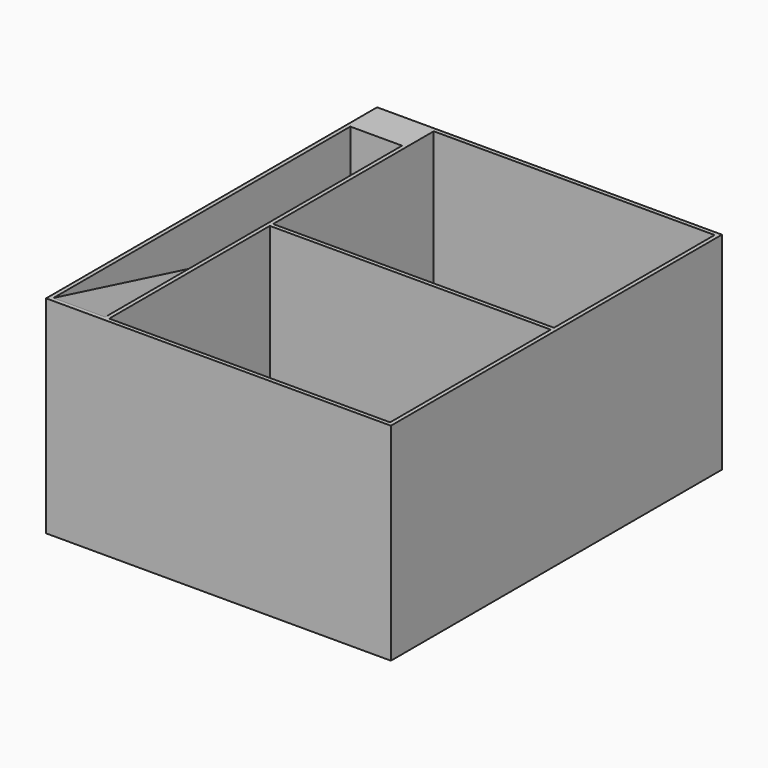
from build123d import *

# Parameters (mm, degrees)
F0_W      = 127
F0_H      = 152.4
F1_DEPTH  = 76.2
F2_T      = -1.4986
F3_W      = 1.4986
F3_H      = 149.4028
F5_DEPTH  = 74.7014
F6_DEPTH  = 19.05
F8_DEPTH  = 19.05
F9_W      = 103.4542
F9_H      = 1.4986
F10_DEPTH = 74.7014


# Not quite as in the source:
# - an extrude ends at something that could not be found from the text; its depth is read off the source's solid


with BuildPart() as f1:
    # F0 (on Top) → F1 (new body)
    with BuildSketch(Plane.XY):
        Rectangle(F0_W, F0_H)
    extrude(amount=F1_DEPTH)

    # F2
    f2_openings = [f1.faces().sort_by_distance(p)[0] for p in [
        (0, 0, 76.2),
    ]]
    offset(amount=F2_T, openings=f2_openings)

    # F3 (on face) → F5 (join, through all)
    with BuildSketch(Plane.XY.offset(1.4986)):
        with Locations((-42.2021, 0)):
            Rectangle(F3_W, F3_H)
    extrude(amount=F5_DEPTH)

    # F4 (on face) → F6 (join, through all)
    with BuildSketch(Plane.YZ.offset(-62.0014)):
        Polygon((-74.7014, 74.7014), (74.7014, 36.6014), (74.7014, 38.1), (-74.7014, 76.2), align=None)
    extrude(amount=F6_DEPTH)

    # F7 (on face) → F8 (join, through all)
    with BuildSketch(Plane(origin=(-42.9514, 0, 0), x_dir=(0, -1, 0), z_dir=(-1, 0, 0))):
        Polygon((-74.7014, 76.2), (-74.7014, 38.1), (-62.0014, 41.3386943217), (-62.0014, 76.2), align=None)
    extrude(amount=F8_DEPTH)

    # F9 (on face) → F10 (join, through all)
    with BuildSketch(Plane.XY.offset(1.4986)):
        with Locations((10.2743, 0)):
            Rectangle(F9_W, F9_H)
    extrude(amount=F10_DEPTH)


solid = f1.part
